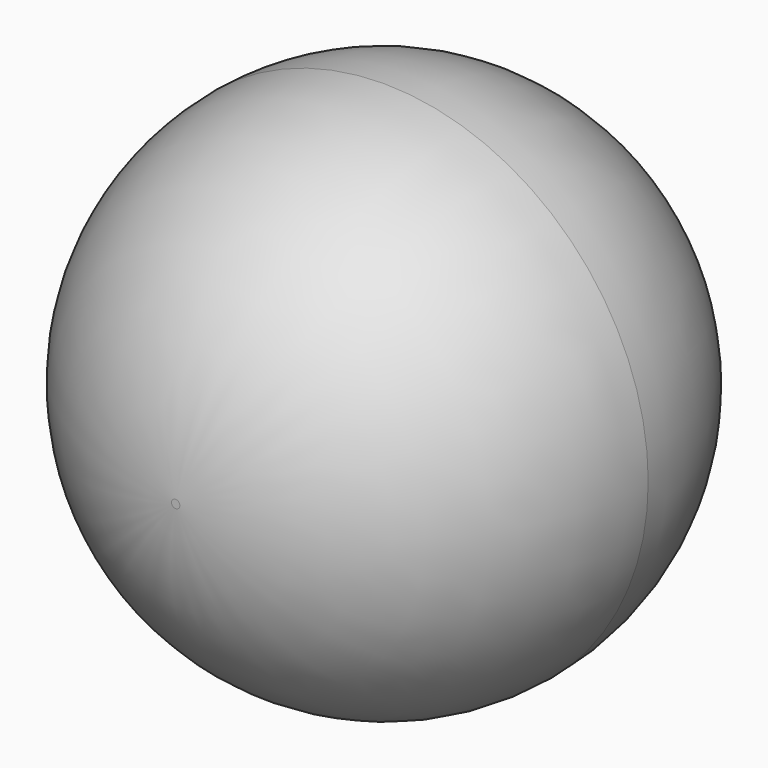
from build123d import *

# Parameters (mm, degrees)
F0_R     = 25.4
F1_DEPTH = 25
F2_R     = 24.99999
F3_DEPTH = 25
F4_R     = 25


# Not quite as in the source:
# - a fillet or chamfer is up to 0.001 mm smaller than in the source, because OpenCascade refuses the exact size


with BuildPart() as f1:
    # F0 (on Front) → F1 (new body)
    with BuildSketch(Plane.XZ):
        Circle(F0_R)
    extrude(amount=-F1_DEPTH)

    # F2 (radius 25 in the source; OpenCascade refuses exactly that, so slightly less here)
    f2_edges = [f1.edges().sort_by_distance(p)[0] for p in [
        (-25.4, 0, 0),
    ]]
    fillet(f2_edges, radius=F2_R)

    # F3 (add): a face of the model
    f3_faces = [f1.faces().sort_by_distance(p)[0] for p in [
        (0, 25, 0),
    ]]
    extrude(f3_faces, amount=F3_DEPTH)

    # F4
    f4_edges = [f1.edges().sort_by_distance(p)[0] for p in [
        (-25.4, 50, 0),
    ]]
    fillet(f4_edges, radius=F4_R)


solid = f1.part
